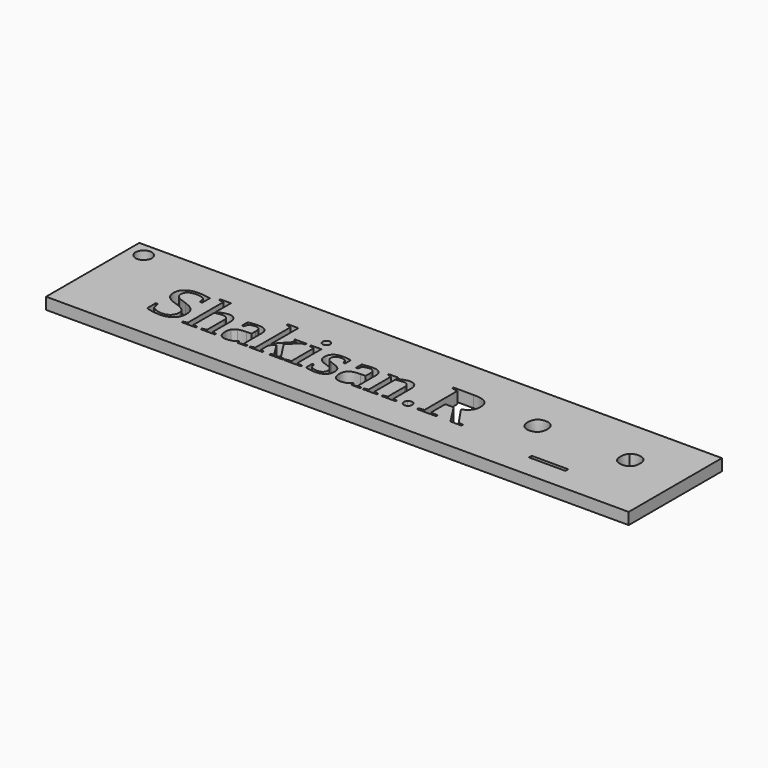
from build123d import *

# Parameters (mm, degrees)
F0_W     = 250
F0_H     = 50
F0_W_2   = 15.6701931701
F0_H_2   = 1.5147853398
F1_DEPTH = 5
F2_R     = 3.5
F3_DEPTH = 25


with BuildPart() as f1:
    # F0 (on Top) → F1 (new body)
    with BuildSketch(Plane.XY):
        with Locations((146.2533682097, 21.8290069513)):
            Rectangle(F0_W, F0_H)
        with BuildLine():
            Line((52.8934113512, 11.4894777835), (52.8934113512, 16.0908163234))
            Line((52.8934113512, 16.0908163234), (53.8621142017, 16.0908163234))
            Line((53.8621142017, 16.0908163234), (54.3797054306, 13.407889311))
            add(Edge.make_bspline(
                [(54.3797054306, 13.407889311), (54.9305364633, 12.7098534334), (56.2719999695, 12.1756423026)],
                knots=[0, 0, 0, 1, 1, 1], degree=2))
            add(Edge.make_bspline(
                [(56.2719999695, 12.1756423026), (57.6134634757, 11.6414311718), (58.9193129066, 11.6414311718)],
                knots=[0, 0, 0, 1, 1, 1], degree=2))
            add(Edge.make_bspline(
                [(58.9193129066, 11.6414311718), (60.9991749091, 11.6414311718), (62.1625680384, 12.7027306183)],
                knots=[0, 0, 0, 1, 1, 1], degree=2))
            add(Edge.make_bspline(
                [(62.1625680384, 12.7027306183), (63.3259611677, 13.7640300648), (63.3259611677, 15.6302076151)],
                knots=[0, 0, 0, 1, 1, 1], degree=2))
            add(Edge.make_bspline(
                [(63.3259611677, 15.6302076151), (63.3259611677, 16.6986298767), (62.8748495462, 17.3966657543)],
                knots=[0, 0, 0, 1, 1, 1], degree=2))
            add(Edge.make_bspline(
                [(62.8748495462, 17.3966657543), (62.4237379246, 18.0947016318), (61.6877136999, 18.5766787854)],
                knots=[0, 0, 0, 1, 1, 1], degree=2))
            add(Edge.make_bspline(
                [(61.6877136999, 18.5766787854), (60.9516894753, 19.058655939), (60.0186007002, 19.3934282476)],
                knots=[0, 0, 0, 1, 1, 1], degree=2))
            add(Edge.make_bspline(
                [(60.0186007002, 19.3934282476), (59.085511925, 19.7282005562), (58.097814901, 20.0700956799)],
                knots=[0, 0, 0, 1, 1, 1], degree=2))
            add(Edge.make_bspline(
                [(58.097814901, 20.0700956799), (57.1101178769, 20.4119908036), (56.1746548301, 20.8274883498)],
                knots=[0, 0, 0, 1, 1, 1], degree=2))
            add(Edge.make_bspline(
                [(56.1746548301, 20.8274883498), (55.2391917833, 21.242985896), (54.5055418303, 21.8792907096)],
                knots=[0, 0, 0, 1, 1, 1], degree=2))
            add(Edge.make_bspline(
                [(54.5055418303, 21.8792907096), (53.7718918774, 22.5155955231), (53.3184059841, 23.458181385)],
                knots=[0, 0, 0, 1, 1, 1], degree=2))
            add(Edge.make_bspline(
                [(53.3184059841, 23.458181385), (52.8649200908, 24.4007672469), (52.8649200908, 25.7825933719)],
                knots=[0, 0, 0, 1, 1, 1], degree=2))
            add(Edge.make_bspline(
                [(52.8649200908, 25.7825933719), (52.8649200908, 28.1568650644), (54.6456238602, 29.5078256574)],
                knots=[0, 0, 0, 1, 1, 1], degree=2))
            add(Edge.make_bspline(
                [(54.6456238602, 29.5078256574), (56.4263276295, 30.8587862504), (59.5888575238, 30.8587862504)],
                knots=[0, 0, 0, 1, 1, 1], degree=2))
            add(Edge.make_bspline(
                [(59.5888575238, 30.8587862504), (61.9916204766, 30.8587862504), (64.8122552472, 30.2177328934)],
                knots=[0, 0, 0, 1, 1, 1], degree=2))
            Line((64.8122552472, 30.2177328934), (64.8122552472, 26.0770030618))
            Line((64.8122552472, 26.0770030618), (63.8483009401, 26.0770030618))
            Line((63.8483009401, 26.0770030618), (63.3259611677, 28.5130058182))
            add(Edge.make_bspline(
                [(63.3259611677, 28.5130058182), (61.8159243713, 29.6099193401), (59.5888575238, 29.6099193401)],
                knots=[0, 0, 0, 1, 1, 1], degree=2))
            add(Edge.make_bspline(
                [(59.5888575238, 29.6099193401), (57.5992178456, 29.6099193401), (56.4785616067, 28.800292693)],
                knots=[0, 0, 0, 1, 1, 1], degree=2))
            add(Edge.make_bspline(
                [(56.4785616067, 28.800292693), (55.3579053679, 27.9906660459), (55.3579053679, 26.5661030304)],
                knots=[0, 0, 0, 1, 1, 1], degree=2))
            add(Edge.make_bspline(
                [(55.3579053679, 26.5661030304), (55.3579053679, 25.6021487233), (55.8113912612, 24.9658439097)],
                knots=[0, 0, 0, 1, 1, 1], degree=2))
            add(Edge.make_bspline(
                [(55.8113912612, 24.9658439097), (56.2648771544, 24.3295390962), (56.9985271074, 23.8760532029)],
                knots=[0, 0, 0, 1, 1, 1], degree=2))
            add(Edge.make_bspline(
                [(56.9985271074, 23.8760532029), (57.7321770603, 23.4225673097), (58.6747629222, 23.0949178161)],
                knots=[0, 0, 0, 1, 1, 1], degree=2))
            add(Edge.make_bspline(
                [(58.6747629222, 23.0949178161), (59.6173487841, 22.7672683225), (60.6050458082, 22.4206246554)],
                knots=[0, 0, 0, 1, 1, 1], degree=2))
            add(Edge.make_bspline(
                [(60.6050458082, 22.4206246554), (61.5927428322, 22.0739809884), (62.5353286941, 21.6347407253)],
                knots=[0, 0, 0, 1, 1, 1], degree=2))
            add(Edge.make_bspline(
                [(62.5353286941, 21.6347407253), (63.477914556, 21.1955004622), (64.211564509, 20.5212073015)],
                knots=[0, 0, 0, 1, 1, 1], degree=2))
            add(Edge.make_bspline(
                [(64.211564509, 20.5212073015), (64.945214462, 19.8469141408), (65.3987003552, 18.8734627469)],
                knots=[0, 0, 0, 1, 1, 1], degree=2))
            add(Edge.make_bspline(
                [(65.3987003552, 18.8734627469), (65.8521862485, 17.900011353), (65.8521862485, 16.4754483376)],
                knots=[0, 0, 0, 1, 1, 1], degree=2))
            add(Edge.make_bspline(
                [(65.8521862485, 16.4754483376), (65.8521862485, 13.5978310464), (64.0857281093, 12.0165660992)],
                knots=[0, 0, 0, 1, 1, 1], degree=2))
            add(Edge.make_bspline(
                [(64.0857281093, 12.0165660992), (62.3192699701, 10.435301152), (58.9952896007, 10.435301152)],
                knots=[0, 0, 0, 1, 1, 1], degree=2))
            add(Edge.make_bspline(
                [(58.9952896007, 10.435301152), (57.3902819366, 10.435301152), (55.7734029141, 10.7178394834)],
                knots=[0, 0, 0, 1, 1, 1], degree=2))
            add(Edge.make_bspline(
                [(55.7734029141, 10.7178394834), (54.1565238915, 11.0003778148), (52.8934113512, 11.4894777835)],
                knots=[0, 0, 0, 1, 1, 1], degree=2))
        make_face(mode=Mode.SUBTRACT)
        with BuildLine():
            Line((72.5713751381, 31.8227405575), (72.5713751381, 25.7825933719))
            add(Edge.make_bspline(
                [(72.5713751381, 25.7825933719), (72.5713751381, 24.2393167719), (72.4669071836, 23.5555265244)],
                knots=[0, 0, 0, 1, 1, 1], degree=2))
            add(Edge.make_bspline(
                [(72.4669071836, 23.5555265244), (73.5353294452, 24.1633400777), (74.8934128533, 24.6097031559)],
                knots=[0, 0, 0, 1, 1, 1], degree=2))
            add(Edge.make_bspline(
                [(74.8934128533, 24.6097031559), (76.2514962613, 25.0560662341), (77.1869593082, 25.0560662341)],
                knots=[0, 0, 0, 1, 1, 1], degree=2))
            add(Edge.make_bspline(
                [(77.1869593082, 25.0560662341), (78.9961543378, 25.0560662341), (79.9149974828, 24.0018896026)],
                knots=[0, 0, 0, 1, 1, 1], degree=2))
            add(Edge.make_bspline(
                [(79.9149974828, 24.0018896026), (80.8338406277, 22.9477129712), (80.8338406277, 20.9438276628)],
                knots=[0, 0, 0, 1, 1, 1], degree=2))
            Line((80.8338406277, 20.9438276628), (80.8338406277, 11.7743903866))
            Line((80.8338406277, 11.7743903866), (82.5290706161, 11.4040040025))
            Line((82.5290706161, 11.4040040025), (82.5290706161, 10.7344593853))
            Line((82.5290706161, 10.7344593853), (76.5174146909, 10.7344593853))
            Line((76.5174146909, 10.7344593853), (76.5174146909, 11.4040040025))
            Line((76.5174146909, 11.4040040025), (78.3740951544, 11.7743903866))
            Line((78.3740951544, 11.7743903866), (78.3740951544, 20.7681315575))
            add(Edge.make_bspline(
                [(78.3740951544, 20.7681315575), (78.3740951544, 23.3180993552), (75.9096011376, 23.3180993552)],
                knots=[0, 0, 0, 1, 1, 1], degree=2))
            add(Edge.make_bspline(
                [(75.9096011376, 23.3180993552), (74.5135293825, 23.3180993552), (72.5713751381, 22.8859819072)],
                knots=[0, 0, 0, 1, 1, 1], degree=2))
            Line((72.5713751381, 22.8859819072), (72.5713751381, 11.7743903866))
            Line((72.5713751381, 11.7743903866), (74.4565468619, 11.4040040025))
            Line((74.4565468619, 11.4040040025), (74.4565468619, 10.7344593853))
            Line((74.4565468619, 10.7344593853), (68.3404229821, 10.7344593853))
            Line((68.3404229821, 10.7344593853), (68.3404229821, 11.4040040025))
            Line((68.3404229821, 11.4040040025), (70.1068811213, 11.7743903866))
            Line((70.1068811213, 11.7743903866), (70.1068811213, 30.7970551864))
            Line((70.1068811213, 30.7970551864), (68.0317676621, 31.1531959402))
            Line((68.0317676621, 31.1531959402), (68.0317676621, 31.8227405575))
            Line((68.0317676621, 31.8227405575), (72.5713751381, 31.8227405575))
        make_face(mode=Mode.SUBTRACT)
        with BuildLine():
            add(Edge.make_bspline(
                [(85.6013781862, 24.4767439411), (88.0041411389, 24.99433517), (89.8275817987, 24.99433517)],
                knots=[0, 0, 0, 1, 1, 1], degree=2))
            add(Edge.make_bspline(
                [(89.8275817987, 24.99433517), (92.1116311668, 24.99433517), (93.1895505152, 24.0588721232)],
                knots=[0, 0, 0, 1, 1, 1], degree=2))
            add(Edge.make_bspline(
                [(93.1895505152, 24.0588721232), (94.2674698636, 23.1234090764), (94.2674698636, 21.1955004622)],
                knots=[0, 0, 0, 1, 1, 1], degree=2))
            Line((94.2674698636, 21.1955004622), (94.2674698636, 11.7743903866))
            Line((94.2674698636, 11.7743903866), (96.000688199, 11.4040040025))
            Line((96.000688199, 11.4040040025), (96.000688199, 10.7344593853))
            Line((96.000688199, 10.7344593853), (92.1733622308, 10.7344593853))
            Line((92.1733622308, 10.7344593853), (91.8931981711, 12.1305311404))
            add(Edge.make_bspline(
                [(91.8931981711, 12.1305311404), (90.1979681827, 10.435301152), (87.5720236909, 10.435301152)],
                knots=[0, 0, 0, 1, 1, 1], degree=2))
            add(Edge.make_bspline(
                [(87.5720236909, 10.435301152), (83.9963705221, 10.435301152), (83.9963705221, 14.5950251572)],
                knots=[0, 0, 0, 1, 1, 1], degree=2))
            add(Edge.make_bspline(
                [(83.9963705221, 14.5950251572), (83.9963705221, 15.9863483689), (84.5377044679, 16.9004429705)],
                knots=[0, 0, 0, 1, 1, 1], degree=2))
            add(Edge.make_bspline(
                [(84.5377044679, 16.9004429705), (85.0790384138, 17.8145375721), (86.26617426, 18.2965147257)],
                knots=[0, 0, 0, 1, 1, 1], degree=2))
            add(Edge.make_bspline(
                [(86.26617426, 18.2965147257), (87.4533101063, 18.7784918793), (89.7088682141, 18.8212287697)],
                knots=[0, 0, 0, 1, 1, 1], degree=2))
            Line((89.7088682141, 18.8212287697), (91.8029758468, 18.8829598337))
            Line((91.8029758468, 18.8829598337), (91.8029758468, 21.0625412474))
            add(Edge.make_bspline(
                [(91.8029758468, 21.0625412474), (91.8029758468, 22.501349893), (91.2758875311, 23.1851401404)],
                knots=[0, 0, 0, 1, 1, 1], degree=2))
            add(Edge.make_bspline(
                [(91.2758875311, 23.1851401404), (90.7487992154, 23.8689303878), (89.6518856935, 23.8689303878)],
                knots=[0, 0, 0, 1, 1, 1], degree=2))
            add(Edge.make_bspline(
                [(89.6518856935, 23.8689303878), (88.165591614, 23.8689303878), (86.9357188773, 23.1708945103)],
                knots=[0, 0, 0, 1, 1, 1], degree=2))
            Line((86.9357188773, 23.1708945103), (86.4323732785, 21.4329276314))
            Line((86.4323732785, 21.4329276314), (85.6013781862, 21.4329276314))
            Line((85.6013781862, 21.4329276314), (85.6013781862, 24.4767439411))
        make_face(mode=Mode.SUBTRACT)
        Polygon((101.5232441556, 31.8227405575), (101.5232441556, 17.4583968183), (107.2357418476, 23.6172575884), (105.7826875719, 24.0161352328), (105.7826875719, 24.68567985), (110.706927062, 24.68567985), (110.706927062, 24.0161352328), (108.9737087265, 23.6742401091), (104.99442937, 19.6094869716), (110.0991135087, 11.7458991263), (111.6138988485, 11.4040040025), (111.6138988485, 10.7344593853), (105.9014011565, 10.7344593853), (105.9014011565, 11.4040040025), (107.178759327, 11.7743903866), (103.3466848154, 17.7812977684), (101.5232441556, 15.7821610034), (101.5232441556, 11.7743903866), (103.0095382351, 11.4040040025), (103.0095382351, 10.7344593853), (97.2922919997, 10.7344593853), (97.2922919997, 11.4040040025), (99.0587501389, 11.7743903866), (99.0587501389, 30.7970551864), (96.9978823099, 31.1531959402), (96.9978823099, 31.8227405575), align=None, mode=Mode.SUBTRACT)
        Polygon((117.0889693713, 24.68567985), (117.0889693713, 11.7743903866), (119.4774866938, 11.4040040025), (119.4774866938, 10.7344593853), (112.2502036621, 10.7344593853), (112.2502036621, 11.4040040025), (114.6244753545, 11.7743903866), (114.6244753545, 23.6457488487), (112.6538298498, 24.0161352328), (112.6538298498, 24.68567985), align=None, mode=Mode.SUBTRACT)
        with BuildLine():
            add(Edge.make_bspline(
                [(130.5249728788, 16.2261498099), (130.7837684932, 15.5874707246), (130.7837684932, 14.6520076778)],
                knots=[0, 0, 0, 1, 1, 1], degree=2))
            add(Edge.make_bspline(
                [(130.7837684932, 14.6520076778), (130.7837684932, 12.5768942186), (129.4707962473, 11.5060976853)],
                knots=[0, 0, 0, 1, 1, 1], degree=2))
            add(Edge.make_bspline(
                [(129.4707962473, 11.5060976853), (128.1578240014, 10.435301152), (125.5936105736, 10.435301152)],
                knots=[0, 0, 0, 1, 1, 1], degree=2))
            add(Edge.make_bspline(
                [(125.5936105736, 10.435301152), (124.5536795723, 10.435301152), (123.3000641187, 10.651359876)],
                knots=[0, 0, 0, 1, 1, 1], degree=2))
            add(Edge.make_bspline(
                [(123.3000641187, 10.651359876), (122.0464486651, 10.8674186001), (121.3341671573, 11.1333370296)],
                knots=[0, 0, 0, 1, 1, 1], degree=2))
            Line((121.3341671573, 11.1333370296), (121.3341671573, 14.5617853535))
            Line((121.3341671573, 14.5617853535), (121.9989632312, 14.5617853535))
            Line((121.9989632312, 14.5617853535), (122.7302389125, 12.6196311091))
            add(Edge.make_bspline(
                [(122.7302389125, 12.6196311091), (123.8413980645, 11.6081913681), (125.6221018339, 11.6081913681)],
                knots=[0, 0, 0, 1, 1, 1], degree=2))
            add(Edge.make_bspline(
                [(125.6221018339, 11.6081913681), (128.4997191251, 11.6081913681), (128.4997191251, 14.0726853848)],
                knots=[0, 0, 0, 1, 1, 1], degree=2))
            add(Edge.make_bspline(
                [(128.4997191251, 14.0726853848), (128.4997191251, 15.8818804145), (126.2299153871, 16.6558929862)],
                knots=[0, 0, 0, 1, 1, 1], degree=2))
            Line((126.2299153871, 16.6558929862), (124.9098203261, 17.0880104342))
            add(Edge.make_bspline(
                [(124.9098203261, 17.0880104342), (123.4092806165, 17.5771104029), (122.7278646408, 18.0804560017)],
                knots=[0, 0, 0, 1, 1, 1], degree=2))
            add(Edge.make_bspline(
                [(122.7278646408, 18.0804560017), (122.0464486651, 18.5838016005), (121.676062281, 19.3198258251)],
                knots=[0, 0, 0, 1, 1, 1], degree=2))
            add(Edge.make_bspline(
                [(121.676062281, 19.3198258251), (121.305675897, 20.0558500498), (121.305675897, 21.0910325077)],
                knots=[0, 0, 0, 1, 1, 1], degree=2))
            add(Edge.make_bspline(
                [(121.305675897, 21.0910325077), (121.305675897, 22.933467341), (122.5592913506, 23.9947667875)],
                knots=[0, 0, 0, 1, 1, 1], degree=2))
            add(Edge.make_bspline(
                [(122.5592913506, 23.9947667875), (123.8129068042, 25.0560662341), (125.9497513274, 25.0560662341)],
                knots=[0, 0, 0, 1, 1, 1], degree=2))
            add(Edge.make_bspline(
                [(125.9497513274, 25.0560662341), (127.4787822974, 25.0560662341), (129.7770772956, 24.5954575257)],
                knots=[0, 0, 0, 1, 1, 1], degree=2))
            Line((129.7770772956, 24.5954575257), (129.7770772956, 21.551641216))
            Line((129.7770772956, 21.551641216), (129.0790414181, 21.551641216))
            Line((129.0790414181, 21.551641216), (128.4569822346, 23.1708945103))
            add(Edge.make_bspline(
                [(128.4569822346, 23.1708945103), (127.6687240327, 23.8689303878), (125.9782425877, 23.8689303878)],
                knots=[0, 0, 0, 1, 1, 1], degree=2))
            add(Edge.make_bspline(
                [(125.9782425877, 23.8689303878), (124.7768611114, 23.8689303878), (124.1453048412, 23.2753624647)],
                knots=[0, 0, 0, 1, 1, 1], degree=2))
            add(Edge.make_bspline(
                [(124.1453048412, 23.2753624647), (123.513748571, 22.6817945416), (123.513748571, 21.6703548006)],
                knots=[0, 0, 0, 1, 1, 1], degree=2))
            add(Edge.make_bspline(
                [(123.513748571, 21.6703548006), (123.513748571, 20.8251140781), (124.0859480489, 20.2457917852)],
                knots=[0, 0, 0, 1, 1, 1], degree=2))
            add(Edge.make_bspline(
                [(124.0859480489, 20.2457917852), (124.6581475267, 19.6664694922), (125.8167921126, 19.281837478)],
                knots=[0, 0, 0, 1, 1, 1], degree=2))
            add(Edge.make_bspline(
                [(125.8167921126, 19.281837478), (127.9963735263, 18.54106471), (128.6635438719, 18.1991695863)],
                knots=[0, 0, 0, 1, 1, 1], degree=2))
            add(Edge.make_bspline(
                [(128.6635438719, 18.1991695863), (129.3307142175, 17.8572744626), (129.7984457409, 17.3610516789)],
                knots=[0, 0, 0, 1, 1, 1], degree=2))
            add(Edge.make_bspline(
                [(129.7984457409, 17.3610516789), (130.2661772643, 16.8648288951), (130.5249728788, 16.2261498099)],
                knots=[0, 0, 0, 1, 1, 1], degree=2))
        make_face(mode=Mode.SUBTRACT)
        with BuildLine():
            add(Edge.make_bspline(
                [(134.5588604842, 24.4767439411), (136.9616234369, 24.99433517), (138.7850640967, 24.99433517)],
                knots=[0, 0, 0, 1, 1, 1], degree=2))
            add(Edge.make_bspline(
                [(138.7850640967, 24.99433517), (141.0691134649, 24.99433517), (142.1470328132, 24.0588721232)],
                knots=[0, 0, 0, 1, 1, 1], degree=2))
            add(Edge.make_bspline(
                [(142.1470328132, 24.0588721232), (143.2249521616, 23.1234090764), (143.2249521616, 21.1955004622)],
                knots=[0, 0, 0, 1, 1, 1], degree=2))
            Line((143.2249521616, 21.1955004622), (143.2249521616, 11.7743903866))
            Line((143.2249521616, 11.7743903866), (144.9581704971, 11.4040040025))
            Line((144.9581704971, 11.4040040025), (144.9581704971, 10.7344593853))
            Line((144.9581704971, 10.7344593853), (141.1308445289, 10.7344593853))
            Line((141.1308445289, 10.7344593853), (140.8506804692, 12.1305311404))
            add(Edge.make_bspline(
                [(140.8506804692, 12.1305311404), (139.1554504808, 10.435301152), (136.5295059889, 10.435301152)],
                knots=[0, 0, 0, 1, 1, 1], degree=2))
            add(Edge.make_bspline(
                [(136.5295059889, 10.435301152), (132.9538528201, 10.435301152), (132.9538528201, 14.5950251572)],
                knots=[0, 0, 0, 1, 1, 1], degree=2))
            add(Edge.make_bspline(
                [(132.9538528201, 14.5950251572), (132.9538528201, 15.9863483689), (133.495186766, 16.9004429705)],
                knots=[0, 0, 0, 1, 1, 1], degree=2))
            add(Edge.make_bspline(
                [(133.495186766, 16.9004429705), (134.0365207119, 17.8145375721), (135.2236565581, 18.2965147257)],
                knots=[0, 0, 0, 1, 1, 1], degree=2))
            add(Edge.make_bspline(
                [(135.2236565581, 18.2965147257), (136.4107924043, 18.7784918793), (138.6663505121, 18.8212287697)],
                knots=[0, 0, 0, 1, 1, 1], degree=2))
            Line((138.6663505121, 18.8212287697), (140.7604581448, 18.8829598337))
            Line((140.7604581448, 18.8829598337), (140.7604581448, 21.0625412474))
            add(Edge.make_bspline(
                [(140.7604581448, 21.0625412474), (140.7604581448, 22.501349893), (140.2333698291, 23.1851401404)],
                knots=[0, 0, 0, 1, 1, 1], degree=2))
            add(Edge.make_bspline(
                [(140.2333698291, 23.1851401404), (139.7062815134, 23.8689303878), (138.6093679915, 23.8689303878)],
                knots=[0, 0, 0, 1, 1, 1], degree=2))
            add(Edge.make_bspline(
                [(138.6093679915, 23.8689303878), (137.123073912, 23.8689303878), (135.8932011753, 23.1708945103)],
                knots=[0, 0, 0, 1, 1, 1], degree=2))
            Line((135.8932011753, 23.1708945103), (135.3898555766, 21.4329276314))
            Line((135.3898555766, 21.4329276314), (134.5588604842, 21.4329276314))
            Line((134.5588604842, 21.4329276314), (134.5588604842, 24.4767439411))
        make_face(mode=Mode.SUBTRACT)
        with Locations((228.2523700111, 7.5743037626)):
            Rectangle(F0_W_2, F0_H_2, mode=Mode.SUBTRACT)
        with BuildLine():
            add(Edge.make_bspline(
                [(165.6451997533, 13.377023779), (166.1651652539, 12.8570582783), (166.1651652539, 12.1020398801)],
                knots=[0, 0, 0, 1, 1, 1], degree=2))
            add(Edge.make_bspline(
                [(166.1651652539, 12.1020398801), (166.1651652539, 11.3707641988), (165.65469684, 10.8365530681)],
                knots=[0, 0, 0, 1, 1, 1], degree=2))
            add(Edge.make_bspline(
                [(165.65469684, 10.8365530681), (165.1442284262, 10.3023419373), (164.3725901261, 10.3023419373)],
                knots=[0, 0, 0, 1, 1, 1], degree=2))
            add(Edge.make_bspline(
                [(164.3725901261, 10.3023419373), (163.6009518261, 10.3023419373), (163.0881091405, 10.8365530681)],
                knots=[0, 0, 0, 1, 1, 1], degree=2))
            add(Edge.make_bspline(
                [(163.0881091405, 10.8365530681), (162.575266455, 11.3707641988), (162.575266455, 12.1020398801)],
                knots=[0, 0, 0, 1, 1, 1], degree=2))
            add(Edge.make_bspline(
                [(162.575266455, 12.1020398801), (162.575266455, 12.8570582783), (163.0952319556, 13.377023779)],
                knots=[0, 0, 0, 1, 1, 1], degree=2))
            add(Edge.make_bspline(
                [(163.0952319556, 13.377023779), (163.6151974562, 13.8969892796), (164.3702158544, 13.8969892796)],
                knots=[0, 0, 0, 1, 1, 1], degree=2))
            add(Edge.make_bspline(
                [(164.3702158544, 13.8969892796), (165.1252342526, 13.8969892796), (165.6451997533, 13.377023779)],
                knots=[0, 0, 0, 1, 1, 1], degree=2))
        make_face(mode=Mode.SUBTRACT)
        with BuildLine():
            Line((150.0486090057, 24.68567985), (150.1863167638, 23.5555265244))
            add(Edge.make_bspline(
                [(150.1863167638, 23.5555265244), (151.3259671762, 24.2108255115), (152.6175709769, 24.6334458728)],
                knots=[0, 0, 0, 1, 1, 1], degree=2))
            add(Edge.make_bspline(
                [(152.6175709769, 24.6334458728), (153.9091747776, 25.0560662341), (154.7686611302, 25.0560662341)],
                knots=[0, 0, 0, 1, 1, 1], degree=2))
            add(Edge.make_bspline(
                [(154.7686611302, 25.0560662341), (156.5778561599, 25.0560662341), (157.4990735765, 24.0018896026)],
                knots=[0, 0, 0, 1, 1, 1], degree=2))
            add(Edge.make_bspline(
                [(157.4990735765, 24.0018896026), (158.4202909932, 22.9477129712), (158.4202909932, 20.9438276628)],
                knots=[0, 0, 0, 1, 1, 1], degree=2))
            Line((158.4202909932, 20.9438276628), (158.4202909932, 11.7743903866))
            Line((158.4202909932, 11.7743903866), (160.1107724382, 11.4040040025))
            Line((160.1107724382, 11.4040040025), (160.1107724382, 10.7344593853))
            Line((160.1107724382, 10.7344593853), (154.1038650563, 10.7344593853))
            Line((154.1038650563, 10.7344593853), (154.1038650563, 11.4040040025))
            Line((154.1038650563, 11.4040040025), (155.9557969764, 11.7743903866))
            Line((155.9557969764, 11.7743903866), (155.9557969764, 20.6779092332))
            add(Edge.make_bspline(
                [(155.9557969764, 20.6779092332), (155.9557969764, 21.9077819699), (155.3551062383, 22.6129406625)],
                knots=[0, 0, 0, 1, 1, 1], degree=2))
            add(Edge.make_bspline(
                [(155.3551062383, 22.6129406625), (154.7544155001, 23.3180993552), (153.4913029597, 23.3180993552)],
                knots=[0, 0, 0, 1, 1, 1], degree=2))
            add(Edge.make_bspline(
                [(153.4913029597, 23.3180993552), (152.1569622685, 23.3180993552), (150.2148080241, 22.8859819072)],
                knots=[0, 0, 0, 1, 1, 1], degree=2))
            Line((150.2148080241, 22.8859819072), (150.2148080241, 11.7743903866))
            Line((150.2148080241, 11.7743903866), (152.0999797479, 11.4040040025))
            Line((152.0999797479, 11.4040040025), (152.0999797479, 10.7344593853))
            Line((152.0999797479, 10.7344593853), (146.0740781925, 10.7344593853))
            Line((146.0740781925, 10.7344593853), (146.0740781925, 11.4040040025))
            Line((146.0740781925, 11.4040040025), (147.7503140074, 11.7743903866))
            Line((147.7503140074, 11.7743903866), (147.7503140074, 23.6457488487))
            Line((147.7503140074, 23.6457488487), (146.0740781925, 24.0161352328))
            Line((146.0740781925, 24.0161352328), (146.0740781925, 24.68567985))
            Line((146.0740781925, 24.68567985), (150.0486090057, 24.68567985))
        make_face(mode=Mode.SUBTRACT)
        with BuildLine():
            Line((178.0365237161, 19.4622821267), (174.4608705473, 19.4622821267))
            Line((174.4608705473, 19.4622821267), (174.4608705473, 11.9215952315))
            Line((174.4608705473, 11.9215952315), (177.4714470533, 11.5227175872))
            Line((177.4714470533, 11.5227175872), (177.4714470533, 10.7344593853))
            Line((177.4714470533, 10.7344593853), (169.2374728239, 10.7344593853))
            Line((169.2374728239, 10.7344593853), (169.2374728239, 11.5227175872))
            Line((169.2374728239, 11.5227175872), (171.5974988862, 11.9215952315))
            Line((171.5974988862, 11.9215952315), (171.5974988862, 29.4627144952))
            Line((171.5974988862, 29.4627144952), (169.0427825451, 29.8473465094))
            Line((169.0427825451, 29.8473465094), (169.0427825451, 30.6356047113))
            Line((169.0427825451, 30.6356047113), (177.6376460718, 30.6356047113))
            add(Edge.make_bspline(
                [(177.6376460718, 30.6356047113), (181.3747497157, 30.6356047113), (183.155453485, 29.3724921709)],
                knots=[0, 0, 0, 1, 1, 1], degree=2))
            add(Edge.make_bspline(
                [(183.155453485, 29.3724921709), (184.9361572543, 28.1093796305), (184.9361572543, 25.3219846636)],
                knots=[0, 0, 0, 1, 1, 1], degree=2))
            add(Edge.make_bspline(
                [(184.9361572543, 25.3219846636), (184.9361572543, 23.3323449853), (183.8534893626, 21.8864135247)],
                knots=[0, 0, 0, 1, 1, 1], degree=2))
            add(Edge.make_bspline(
                [(183.8534893626, 21.8864135247), (182.7708214708, 20.440482064), (180.8571584867, 19.8754054012)],
                knots=[0, 0, 0, 1, 1, 1], degree=2))
            Line((180.8571584867, 19.8754054012), (186.2420066852, 11.9215952315))
            Line((186.2420066852, 11.9215952315), (188.3930968385, 11.5227175872))
            Line((188.3930968385, 11.5227175872), (188.3930968385, 10.7344593853))
            Line((188.3930968385, 10.7344593853), (183.6303078235, 10.7344593853))
            Line((183.6303078235, 10.7344593853), (178.0365237161, 19.4622821267))
        make_face(mode=Mode.SUBTRACT)
        with BuildLine():
            add(Edge.make_bspline(
                [(116.7613198777, 30.3839319119), (117.2361742162, 29.9090775734), (117.2361742162, 29.2395329561)],
                knots=[0, 0, 0, 1, 1, 1], degree=2))
            add(Edge.make_bspline(
                [(117.2361742162, 29.2395329561), (117.2361742162, 28.584233969), (116.7613198777, 28.1093796305)],
                knots=[0, 0, 0, 1, 1, 1], degree=2))
            add(Edge.make_bspline(
                [(116.7613198777, 28.1093796305), (116.2864655392, 27.634525292), (115.6216694653, 27.634525292)],
                knots=[0, 0, 0, 1, 1, 1], degree=2))
            add(Edge.make_bspline(
                [(115.6216694653, 27.634525292), (114.9663704782, 27.634525292), (114.4915161397, 28.1093796305)],
                knots=[0, 0, 0, 1, 1, 1], degree=2))
            add(Edge.make_bspline(
                [(114.4915161397, 28.1093796305), (114.0166618012, 28.584233969), (114.0166618012, 29.2395329561)],
                knots=[0, 0, 0, 1, 1, 1], degree=2))
            add(Edge.make_bspline(
                [(114.0166618012, 29.2395329561), (114.0166618012, 29.9090775734), (114.4915161397, 30.3839319119)],
                knots=[0, 0, 0, 1, 1, 1], degree=2))
            add(Edge.make_bspline(
                [(114.4915161397, 30.3839319119), (114.9663704782, 30.8587862504), (115.6216694653, 30.8587862504)],
                knots=[0, 0, 0, 1, 1, 1], degree=2))
            add(Edge.make_bspline(
                [(115.6216694653, 30.8587862504), (116.2864655392, 30.8587862504), (116.7613198777, 30.3839319119)],
                knots=[0, 0, 0, 1, 1, 1], degree=2))
        make_face(mode=Mode.SUBTRACT)
        with BuildLine():
            add(Edge.make_bspline(
                [(211.4282807985, 29.7879897171), (212.5109486903, 28.6317194029), (212.5109486903, 26.5993428341)],
                knots=[0, 0, 0, 1, 1, 1], degree=2))
            add(Edge.make_bspline(
                [(212.5109486903, 26.5993428341), (212.5109486903, 24.4482526808), (211.4116608967, 23.303853725)],
                knots=[0, 0, 0, 1, 1, 1], degree=2))
            add(Edge.make_bspline(
                [(211.4116608967, 23.303853725), (210.3123731031, 22.1594547693), (208.2799965344, 22.1594547693)],
                knots=[0, 0, 0, 1, 1, 1], degree=2))
            add(Edge.make_bspline(
                [(208.2799965344, 22.1594547693), (206.3663335502, 22.1594547693), (205.2765428434, 23.3109765401)],
                knots=[0, 0, 0, 1, 1, 1], degree=2))
            add(Edge.make_bspline(
                [(205.2765428434, 23.3109765401), (204.1867521366, 24.4624983109), (204.1867521366, 26.5993428341)],
                knots=[0, 0, 0, 1, 1, 1], degree=2))
            add(Edge.make_bspline(
                [(204.1867521366, 26.5993428341), (204.1867521366, 28.7361873573), (205.2907884736, 29.8402236943)],
                knots=[0, 0, 0, 1, 1, 1], degree=2))
            add(Edge.make_bspline(
                [(205.2907884736, 29.8402236943), (206.3948248106, 30.9442600313), (208.3702188587, 30.9442600313)],
                knots=[0, 0, 0, 1, 1, 1], degree=2))
            add(Edge.make_bspline(
                [(208.3702188587, 30.9442600313), (210.3456129068, 30.9442600313), (211.4282807985, 29.7879897171)],
                knots=[0, 0, 0, 1, 1, 1], degree=2))
        make_face(mode=Mode.SUBTRACT)
        with BuildLine():
            add(Edge.make_bspline(
                [(251.2400685373, 29.7879897171), (252.3227364291, 28.6317194029), (252.3227364291, 26.5993428341)],
                knots=[0, 0, 0, 1, 1, 1], degree=2))
            add(Edge.make_bspline(
                [(252.3227364291, 26.5993428341), (252.3227364291, 24.4482526808), (251.2234486355, 23.303853725)],
                knots=[0, 0, 0, 1, 1, 1], degree=2))
            add(Edge.make_bspline(
                [(251.2234486355, 23.303853725), (250.1241608419, 22.1594547693), (248.0917842731, 22.1594547693)],
                knots=[0, 0, 0, 1, 1, 1], degree=2))
            add(Edge.make_bspline(
                [(248.0917842731, 22.1594547693), (246.178121289, 22.1594547693), (245.0883305822, 23.3109765401)],
                knots=[0, 0, 0, 1, 1, 1], degree=2))
            add(Edge.make_bspline(
                [(245.0883305822, 23.3109765401), (243.9985398754, 24.4624983109), (243.9985398754, 26.5993428341)],
                knots=[0, 0, 0, 1, 1, 1], degree=2))
            add(Edge.make_bspline(
                [(243.9985398754, 26.5993428341), (243.9985398754, 28.7361873573), (245.1025762124, 29.8402236943)],
                knots=[0, 0, 0, 1, 1, 1], degree=2))
            add(Edge.make_bspline(
                [(245.1025762124, 29.8402236943), (246.2066125493, 30.9442600313), (248.1820065974, 30.9442600313)],
                knots=[0, 0, 0, 1, 1, 1], degree=2))
            add(Edge.make_bspline(
                [(248.1820065974, 30.9442600313), (250.1574006455, 30.9442600313), (251.2400685373, 29.7879897171)],
                knots=[0, 0, 0, 1, 1, 1], degree=2))
        make_face(mode=Mode.SUBTRACT)
    extrude(amount=F1_DEPTH)

    # F2 (on face) → F3 (cut)
    with BuildSketch(Plane.XY.offset(5)):
        with Locations((27.9994625598, 40.7568439841)):
            Circle(F2_R)
    extrude(amount=-F3_DEPTH, mode=Mode.SUBTRACT)


solid = f1.part
